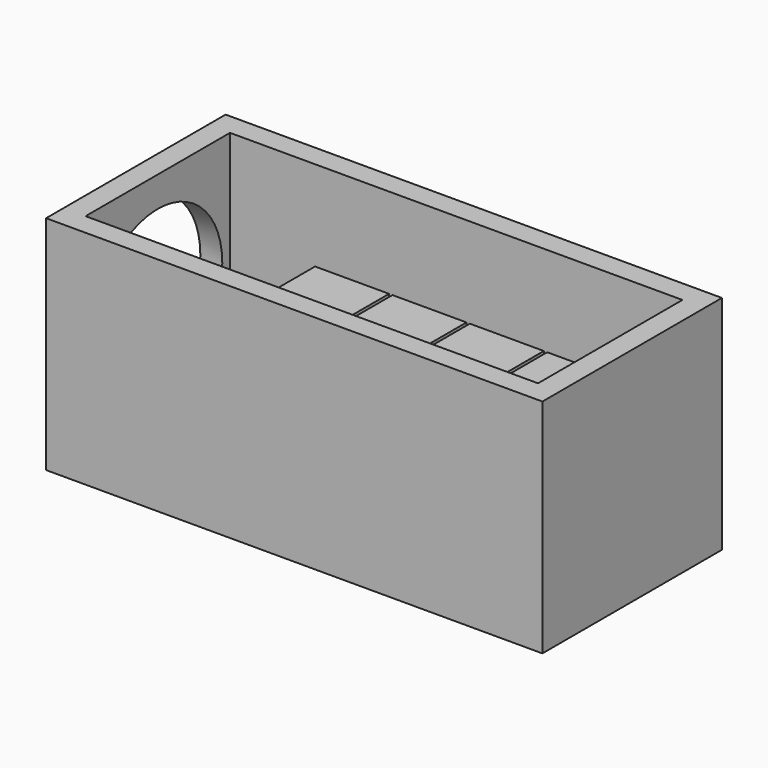
from build123d import *

# Parameters (mm, degrees)
F0_W      = 64.262
F0_H      = 150.876
F1_DEPTH  = 97.282
F2_W      = 64.262
F2_H      = 150.876
F3_DEPTH  = 97.282
F4_W      = 64.262
F4_H      = 150.876
F5_DEPTH  = 97.282
F6_W      = 64.262
F6_H      = 150.876
F7_DEPTH  = 97.282
F8_W      = 392.8110076251
F8_H      = 156.718
F9_DEPTH  = 173.482
F10_T     = 19.05
F12_D     = 139.999974
F12_DEPTH = 25.4
F12_TIP   = 42.0602355207


with BuildPart() as f1:
    # F0 (on Top) → F1 (new body)
    with BuildSketch(Plane.XY):
        Rectangle(F0_W, F0_H)
    extrude(amount=F1_DEPTH)


with BuildPart() as f3:
    # F2 (on Top) → F3 (new body)
    with BuildSketch(Plane.XY):
        with Locations((-67.183, 0)):
            Rectangle(F2_W, F2_H)
    extrude(amount=F3_DEPTH)


with BuildPart() as f5:
    # F4 (on Top) → F5 (new body)
    with BuildSketch(Plane.XY):
        with Locations((67.1830076251, 0)):
            Rectangle(F4_W, F4_H)
    extrude(amount=F5_DEPTH)


with BuildPart() as f7:
    # F6 (on Top) → F7 (new body)
    with BuildSketch(Plane.XY):
        with Locations((134.3660076251, 0)):
            Rectangle(F6_W, F6_H)
    extrude(amount=F7_DEPTH)


with BuildPart() as f9:
    # F8 (on Top) → F9 (new body)
    with BuildSketch(Plane.XY):
        with Locations((20.8915038126, 0)):
            Rectangle(F8_W, F8_H)
    extrude(amount=F9_DEPTH)

    # F10
    f10_openings = [f9.faces().sort_by_distance(p)[0] for p in [
        (20.891504, 0, 173.482),
    ]]
    offset(amount=F10_T, openings=f10_openings, kind=Kind.INTERSECTION)

    # F12
    with Locations(Plane(origin=(-194.564, 0, 0), x_dir=(0, -1, 0), z_dir=(-1, 0, 0))):
        with Locations((0, 77.216)):
            Hole(F12_D / 2, depth=F12_DEPTH)
            with Locations((0, 0, -(F12_DEPTH + F12_TIP / 2))):  # 118° drill point
                Cone(0, F12_D / 2, F12_TIP, mode=Mode.SUBTRACT)


solid = Compound([f1.part, f3.part, f5.part, f7.part, f9.part])
